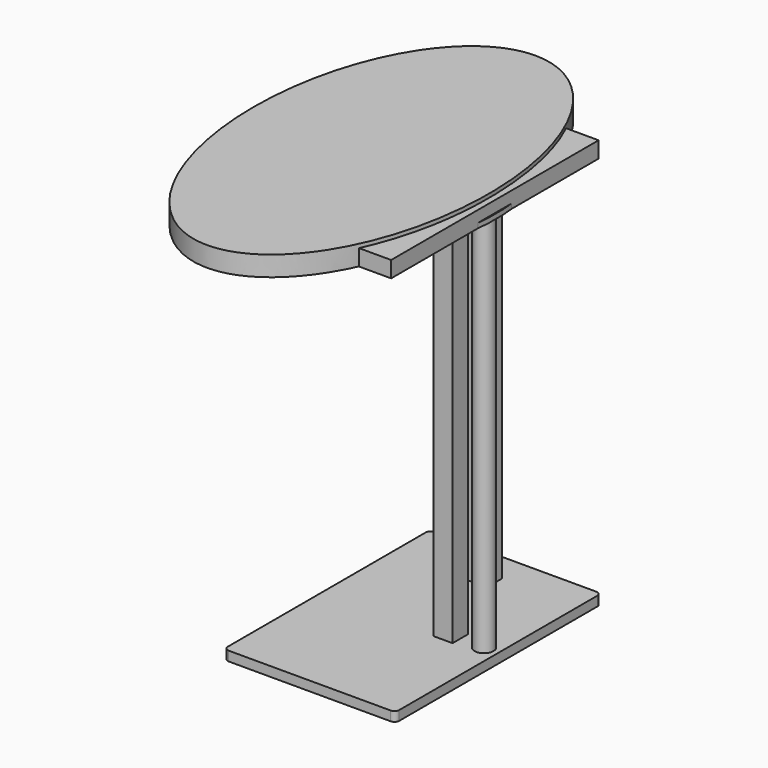
from build123d import *

# Parameters (mm, degrees)
F0_W      = 180
F0_H      = 270
F1_DEPTH  = 10
F2_R      = 5
F3_R      = 10
F4_DEPTH  = 400
F8_DEPTH  = 21
F11_W     = 178.5603770986
F11_H     = 272.1895948052
F11_R     = 10
F12_DEPTH = 17
F18_W     = 20
F18_H     = 20
F19_DEPTH = 400
F23_START = -15
F23_DEPTH = 5
F24_W     = 20
F24_H     = 20
F25_DEPTH = 400


# Not quite as in the source:
# - the program builds the solid bodies; features that only make, move or delete a surface that nothing else refers to are left out


with BuildPart() as f1:
    # F0 (on Top) → F1 (new body)
    with BuildSketch(Plane.XY):
        with Locations((-90, 0)):
            Rectangle(F0_W, F0_H)
    extrude(amount=F1_DEPTH)

    # F2
    f2_edges = [f1.edges().sort_by_distance(p)[0] for p in [
        (-180, -135, 5),
        (0, -135, 5),
        (-180, 135, 5),
        (0, 135, 5),
    ]]
    fillet(f2_edges, radius=F2_R)


with BuildPart() as f4:
    # F3 (on face) → F4 (new body)
    with BuildSketch(Plane.XY.offset(10)):
        with Locations((-15, 0)):
            Circle(F3_R)
    extrude(amount=F4_DEPTH)


with BuildPart() as f8:
    # F7 (on face) → F8 (new body)
    with BuildSketch(Plane.XY.offset(410)):
        with BuildLine():
            ThreePointArc((-10.0412616183, 8.6839457427), (-25, 0), (-10.0412616183, -8.6839457427))
            add(Edge.make_bspline(
                [(-10.0412616183, -8.6839457427), (-9.8405786461, 0), (-10.0412616183, 8.6839457427)],
                knots=[1.5304787343, 1.5304787343, 1.5304787343, 1.6111139193, 1.6111139193, 1.6111139193], degree=2, weights=[1, 0.999187356, 1]))
        make_face()
        with BuildLine():
            add(Edge.make_bspline(
                [(-10.0412616183, 8.6839457427), (-21.7173481471, 513.9311064222), (-222.3823430066, 149.2421217958), (-423.0473378661, -215.4468628305), (-133.3660930395, -215.4468628305)],
                knots=[1.6111139193, 1.6111139193, 1.6111139193, 3.9471496133, 3.9471496133, 6.2831853072, 6.2831853072, 6.2831853072], degree=2, weights=[1, 0.3919759853, 1, 0.3919759853, 1]))
            add(Edge.make_bspline(
                [(-133.3660930395, -215.4468628305), (-14.8194808717, -215.4468628305), (-10.0412616183, -8.6839457427)],
                knots=[0, 0, 0, 1.5304787343, 1.5304787343, 1.5304787343], degree=2, weights=[1, 0.7212165662, 1]))
            ThreePointArc((-10.0412616183, -8.6839457427), (-25, 0), (-10.0412616183, 8.6839457427))
        make_face()
    extrude(amount=F8_DEPTH)


with BuildPart() as f12:
    # F11 (on face) → F12 (new body)
    with BuildSketch(Plane.XY.offset(410)):
        with Locations((-93.1087951176, 0.2716593444)):
            Rectangle(F11_W, F11_H)
        with Locations((-15, 0)):
            Circle(F11_R, mode=Mode.SUBTRACT)
        with Locations((-15, 0)):
            Circle(F11_R)
    extrude(amount=F12_DEPTH)


with BuildPart() as f19:
    # F18 (on face) → F19 (new body)
    with BuildSketch(Plane.XY.offset(10)):
        with Locations((-50, 0)):
            Rectangle(F18_W, F18_H)
    extrude(amount=F19_DEPTH)


with BuildPart() as f23:
    # F22 (on offset) → F23 (new body)
    with BuildSketch(Plane.XY.offset(430).offset(F23_START)):
        with BuildLine():
            add(Edge.make_bspline(
                [(-90, -137.5), (61.5544456623, -137.5), (-14.2227771689, 68.75), (-90, 275), (-165.7772228311, 68.75), (-241.5544456623, -137.5), (-90, -137.5)],
                knots=[0, 0, 0, 2.0943951024, 2.0943951024, 4.1887902048, 4.1887902048, 6.2831853072, 6.2831853072, 6.2831853072], degree=2, weights=[1, 0.5, 1, 0.5, 1, 0.5, 1]))
        make_face()
    extrude(amount=-F23_DEPTH)


with BuildPart() as f25:
    # F24 (on face) → F25 (new body)
    with BuildSketch(Plane.XY.offset(10)):
        with Locations((-90, 95)):
            Rectangle(F24_W, F24_H)
    extrude(amount=F25_DEPTH)


solid = Compound([f1.part, f4.part, f8.part, f12.part, f19.part, f23.part, f25.part])
